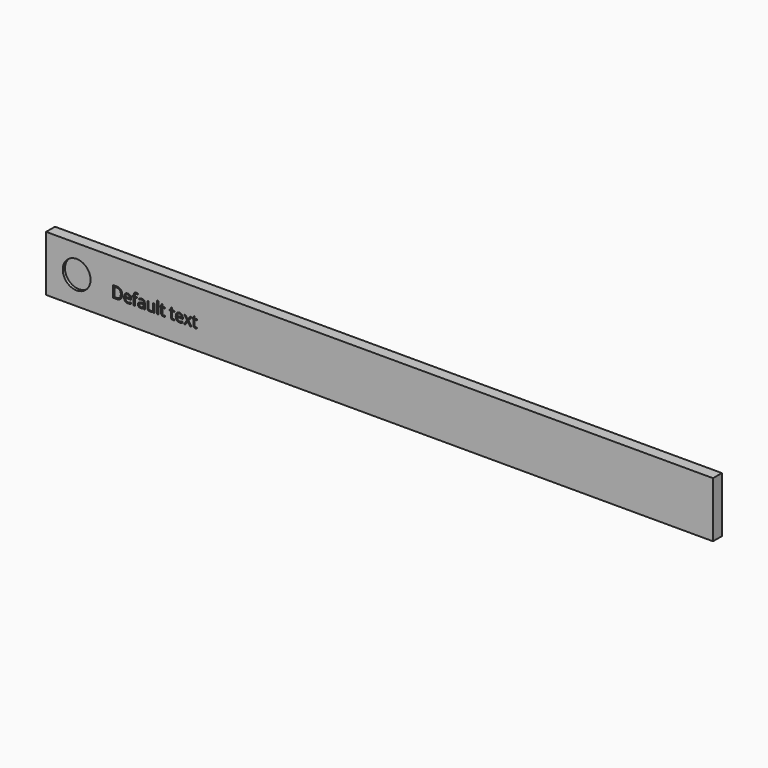
from build123d import *

# Parameters (mm, degrees)
F1_W         = 120
F1_H         = 10
F2_DEPTH     = 2
F3_R         = 2.5
F3_TEXT_SIZE = 2.8292144028
F4_DEPTH     = 0.5


# Not quite as in the source:
# - Text() gives the source's letters only with a copy of the font that has no kerning and outlines rounded to 1/6400 em; it was checked with that copy


with BuildPart() as f2:
    # F1 (on face) → F2 (new body)
    with BuildSketch(Plane.XZ):
        with Locations((4.8347301781, -5.9943100051)):
            Rectangle(F1_W, F1_H)
    extrude(amount=F2_DEPTH)

    # F3 (on face) → F4 (cut)
    with BuildSketch(Plane.XZ.offset(2)):
        with Locations((-49.6652698219, -5.9943100051)):
            Circle(F3_R)
        with Locations((-43.3620475233, -7.5239310972)):
            Text('Default text', F3_TEXT_SIZE, font='Open Sans', text_align=(TextAlign.LEFT, TextAlign.BOTTOM))
    extrude(amount=-F4_DEPTH, mode=Mode.SUBTRACT)


solid = f2.part
